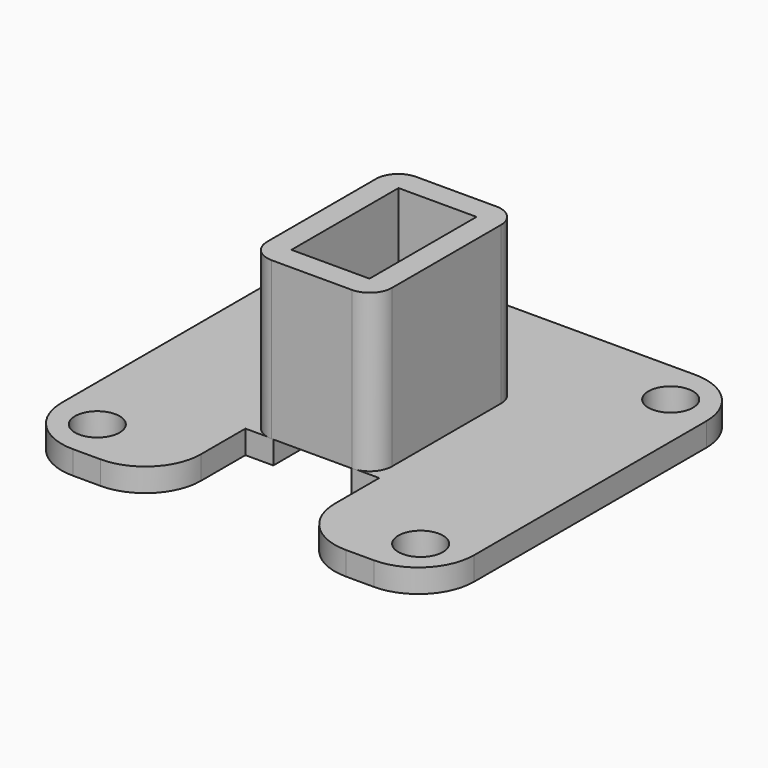
from build123d import *

# Parameters (mm, degrees)
F0_W        = 11.2
F0_H        = 16.2
F0_W_2      = 7
F0_H_2      = 12
F1_DEPTH    = 14.1
F2_R        = 2
F3_DEPTH    = 2.1
F4_R        = 5
F5_T1_DEPTH = 19.1


# Not quite as in the source:
# - a fillet or chamfer that OpenCascade refuses, or shapes differently, is made with other operations: its cross-section is extruded or revolved along the edge and cut away or added


with BuildPart() as f1:
    # F0 (on Top) → F1 (new body)
    with BuildSketch(Plane.XY):
        Rectangle(F0_W, F0_H)
        Rectangle(F0_W_2, F0_H_2, mode=Mode.SUBTRACT)
    extrude(amount=F1_DEPTH)

    # F2 (on Top) → F3 (join)
    with BuildSketch(Plane.XY):
        Polygon((6, -18.0165283297), (18.5, -18.0165283297), (18.5, 0), (18.5, 18.0165283297), (-18.5, 18.0165283297), (-18.5, 0), (-18.5, -14.0165283297), (-18.5, -18.0165283297), (-14.5, -18.0165283297), (-6, -18.0165283297), (-6, -8.0361003056), (-3.5, -8.0361003056), (-3.5, -6), (-3.5, 0), (-3.5, 6), (3.5, 6), (3.5, 0), (3.5, -6), (3.5, -8.0361003056), (6, -8.0361003056), align=None)
        with Locations((-14.5, -14.0165283297)):
            Circle(F2_R, mode=Mode.SUBTRACT)
        with Locations((14.5, -14.0165283297)):
            Circle(F2_R, mode=Mode.SUBTRACT)
        with Locations((-14.5, 14.0165283297)):
            Circle(F2_R, mode=Mode.SUBTRACT)
        with Locations((14.5, 14.0165283297)):
            Circle(F2_R, mode=Mode.SUBTRACT)
    extrude(amount=-F3_DEPTH)

    # F4
    f4_edges = [f1.edges().sort_by_distance(p)[0] for p in [
        (-18.5, 18.016528, -1.05),
        (18.5, 18.016528, -1.05),
        (18.5, -18.016528, -1.05),
        (-18.5, -18.016528, -1.05),
        (6, -18.016528, -1.05),
        (-6, -18.016528, -1.05),
    ]]
    fillet(f4_edges, radius=F4_R)

    # F5: fillet of radius 2 on 4 edges, made by hand

    # F5_s2 → F5_t1 (cut)
    with BuildSketch(Plane.XY):
        with BuildLine():
            ThreePointArc((5.6, 6.1), (5.0142135624, 7.5142135624), (3.6, 8.1))
            Line((3.6, 8.1), (5.6, 8.1))
            Line((5.6, 8.1), (5.6, 6.1))
        make_face()
        with BuildLine():
            ThreePointArc((-3.6, 8.1), (-5.0142135624, 7.5142135624), (-5.6, 6.1))
            Line((-5.6, 6.1), (-5.6, 8.1))
            Line((-5.6, 8.1), (-3.6, 8.1))
        make_face()
        with BuildLine():
            ThreePointArc((5.6, -6.1), (5.0142135624, -7.5142135624), (3.6, -8.1))
            Line((3.6, -8.1), (5.6, -8.1))
            Line((5.6, -8.1), (5.6, -6.1))
        make_face()
        with BuildLine():
            ThreePointArc((-5.6, -6.1), (-5.0142135624, -7.5142135624), (-3.6, -8.1))
            Line((-3.6, -8.1), (-5.6, -8.1))
            Line((-5.6, -8.1), (-5.6, -6.1))
        make_face()
    extrude(amount=F5_T1_DEPTH, mode=Mode.SUBTRACT)


solid = f1.part
